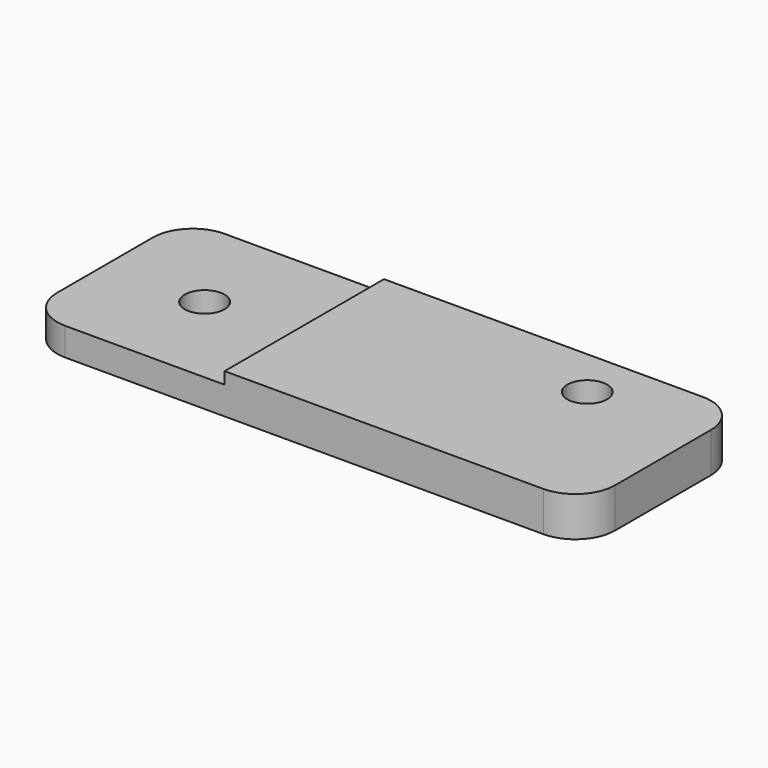
from build123d import *

# Parameters (mm, degrees)
F1_DEPTH = 50
F2_R     = 10
F3_R     = 5
F4_DEPTH = 25


# Not quite as in the source:
# - a feature of the source that left no trace in its solid (it failed there, or was rolled back) is left out


with BuildPart() as f1:
    # F0 (on Front) → F1 (new body)
    with BuildSketch(Plane.XZ):
        Polygon((50, 0), (0, 0), (0, -7), (140, -7), (140, 3), (50, 3), align=None)
    extrude(amount=F1_DEPTH)

    # F2
    f2_edges = [f1.edges().sort_by_distance(p)[0] for p in [
        (0, -50, -3.5),
        (0, 0, -3.5),
        (140, 0, -2),
        (140, -50, -2),
    ]]
    fillet(f2_edges, radius=F2_R)

    # F3 (on face) → F4 (cut)
    with BuildSketch(Plane(origin=(0, 0, -7), x_dir=(1, 0, 0), z_dir=(0, 0, -1))):
        with Locations((25, 25)):
            Circle(F3_R)
        with Locations((111.0006011832, 12.5048019411)):
            Circle(F3_R)
    extrude(amount=-F4_DEPTH, mode=Mode.SUBTRACT)


solid = f1.part
